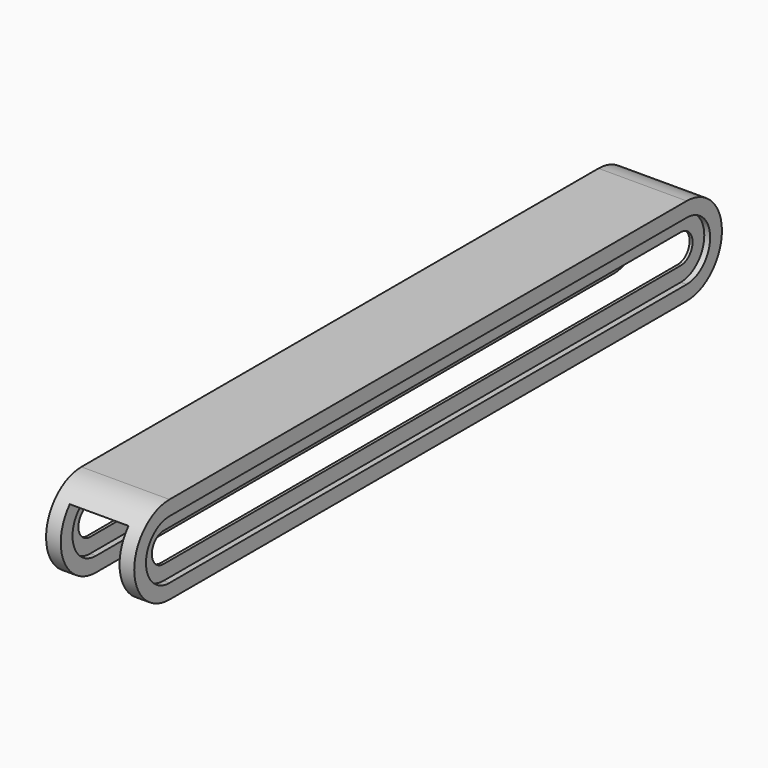
from build123d import *

# Parameters (mm, degrees)
F1_DEPTH      = 125
F1_DEPTH_BACK = 125
F6_DEPTH      = 5.001
F7_DEPTH      = 5.001
F8_DEPTH      = 2
F9_DEPTH      = 2
F10_DEPTH     = 2
F11_DEPTH     = 2
F12_T1_DEPTH  = 80
F12_T3_DEPTH  = 80
F12_T5_DEPTH  = 105


# Not quite as in the source:
# - a fillet or chamfer that OpenCascade refuses, or shapes differently, is made with other operations: its cross-section is extruded or revolved along the edge and cut away or added


with BuildPart() as f1:
    # F0 (on Front) → F1 (new body, two sides)
    with BuildSketch(Plane.XZ) as f1_sk:
        Polygon((15, -15), (15, 15), (-15, 15), (-15, -15), (-10, -15), (-10, 10), (10, 10), (10, -15), align=None)
    extrude(amount=F1_DEPTH)
    extrude(f1_sk.sketch, amount=-F1_DEPTH_BACK)

    # F2 (on face) → F6 (cut, through all)
    with BuildSketch(Plane(origin=(10, 0, 0), x_dir=(0, -1, 0), z_dir=(-1, 0, 0))):
        with BuildLine():
            Line((-110, -5), (110, -5))
            ThreePointArc((110, -5), (115, 0), (110, 5))
            Line((110, 5), (-110, 5))
            ThreePointArc((-110, 5), (-115, 0), (-110, -5))
        make_face()
    extrude(amount=-F6_DEPTH, mode=Mode.SUBTRACT)

    # F4 (on face) → F7 (cut, through all)
    with BuildSketch(Plane.YZ.offset(-10)):
        with BuildLine():
            Line((110, 5), (-110, 5))
            ThreePointArc((-110, 5), (-115, 0), (-110, -5))
            Line((-110, -5), (110, -5))
            ThreePointArc((110, -5), (115, 0), (110, 5))
        make_face()
    extrude(amount=-F7_DEPTH, mode=Mode.SUBTRACT)

    # F2 (on face) → F8 (cut)
    with BuildSketch(Plane(origin=(10, 0, 0), x_dir=(0, -1, 0), z_dir=(-1, 0, 0))):
        with BuildLine():
            Line((-110, -10), (110, -10))
            ThreePointArc((110, -10), (120, 0), (110, 10))
            Line((110, 10), (-110, 10))
            ThreePointArc((-110, 10), (-120, 0), (-110, -10))
        make_face()
        with BuildLine():
            ThreePointArc((110, 5), (115, 0), (110, -5))
            Line((110, -5), (-110, -5))
            ThreePointArc((-110, -5), (-115, 0), (-110, 5))
            Line((-110, 5), (110, 5))
        make_face(mode=Mode.SUBTRACT)
    extrude(amount=-F8_DEPTH, mode=Mode.SUBTRACT)

    # F3 (on face) → F9 (cut)
    with BuildSketch(Plane.YZ.offset(15)):
        with BuildLine():
            ThreePointArc((-110, 10), (-120, 0), (-110, -10))
            Line((-110, -10), (110, -10))
            ThreePointArc((110, -10), (120, 0), (110, 10))
            Line((110, 10), (-110, 10))
        make_face()
        with BuildLine():
            ThreePointArc((-110, -5), (-115, 0), (-110, 5))
            Line((-110, 5), (110, 5))
            ThreePointArc((110, 5), (115, 0), (110, -5))
            Line((110, -5), (-110, -5))
        make_face(mode=Mode.SUBTRACT)
    extrude(amount=-F9_DEPTH, mode=Mode.SUBTRACT)

    # F5 (on face) → F10 (cut)
    with BuildSketch(Plane(origin=(-15, 0, 0), x_dir=(0, -1, 0), z_dir=(-1, 0, 0))):
        with BuildLine():
            Line((110, 10), (-110, 10))
            ThreePointArc((-110, 10), (-120, 0), (-110, -10))
            Line((-110, -10), (110, -10))
            ThreePointArc((110, -10), (120, 0), (110, 10))
        make_face()
        with BuildLine():
            ThreePointArc((-110, -5), (-115, 0), (-110, 5))
            Line((-110, 5), (110, 5))
            ThreePointArc((110, 5), (115, 0), (110, -5))
            Line((110, -5), (-110, -5))
        make_face(mode=Mode.SUBTRACT)
    extrude(amount=-F10_DEPTH, mode=Mode.SUBTRACT)

    # F4 (on face) → F11 (cut)
    with BuildSketch(Plane.YZ.offset(-10)):
        with BuildLine():
            Line((110, 10), (-110, 10))
            ThreePointArc((-110, 10), (-120, 0), (-110, -10))
            Line((-110, -10), (110, -10))
            ThreePointArc((110, -10), (120, 0), (110, 10))
        make_face()
        with BuildLine():
            ThreePointArc((-110, -5), (-115, 0), (-110, 5))
            Line((-110, 5), (110, 5))
            ThreePointArc((110, 5), (115, 0), (110, -5))
            Line((110, -5), (-110, -5))
        make_face(mode=Mode.SUBTRACT)
    extrude(amount=-F11_DEPTH, mode=Mode.SUBTRACT)

    # F12: fillet of radius 15 on 6 edges, made by hand

    # F12_s2 → F12_t1 (cut)
    with BuildSketch(Plane.YZ.offset(-52.5)):
        with BuildLine():
            ThreePointArc((125, 0), (120.6066017178, -10.6066017178), (110, -15))
            Line((110, -15), (125, -15))
            Line((125, -15), (125, 0))
        make_face()
        with BuildLine():
            ThreePointArc((-125, 0), (-120.6066017178, -10.6066017178), (-110, -15))
            Line((-110, -15), (-125, -15))
            Line((-125, -15), (-125, 0))
        make_face()
    extrude(amount=F12_T1_DEPTH, mode=Mode.SUBTRACT)

    # F12_s4 → F12_t3 (cut)
    with BuildSketch(Plane.YZ.offset(-27.5)):
        with BuildLine():
            ThreePointArc((110, -15), (120.6066017178, -10.6066017178), (125, 0))
            Line((125, 0), (125, -15))
            Line((125, -15), (110, -15))
        make_face()
        with BuildLine():
            ThreePointArc((-110, -15), (-120.6066017178, -10.6066017178), (-125, 0))
            Line((-125, 0), (-125, -15))
            Line((-125, -15), (-110, -15))
        make_face()
    extrude(amount=F12_T3_DEPTH, mode=Mode.SUBTRACT)

    # F12_s6 → F12_t5 (cut)
    with BuildSketch(Plane.YZ.offset(-52.5)):
        with BuildLine():
            ThreePointArc((125, 0), (120.6066017178, 10.6066017178), (110, 15))
            Line((110, 15), (125, 15))
            Line((125, 15), (125, 0))
        make_face()
        with BuildLine():
            ThreePointArc((-125, 0), (-120.6066017178, 10.6066017178), (-110, 15))
            Line((-110, 15), (-125, 15))
            Line((-125, 15), (-125, 0))
        make_face()
    extrude(amount=F12_T5_DEPTH, mode=Mode.SUBTRACT)


solid = f1.part
